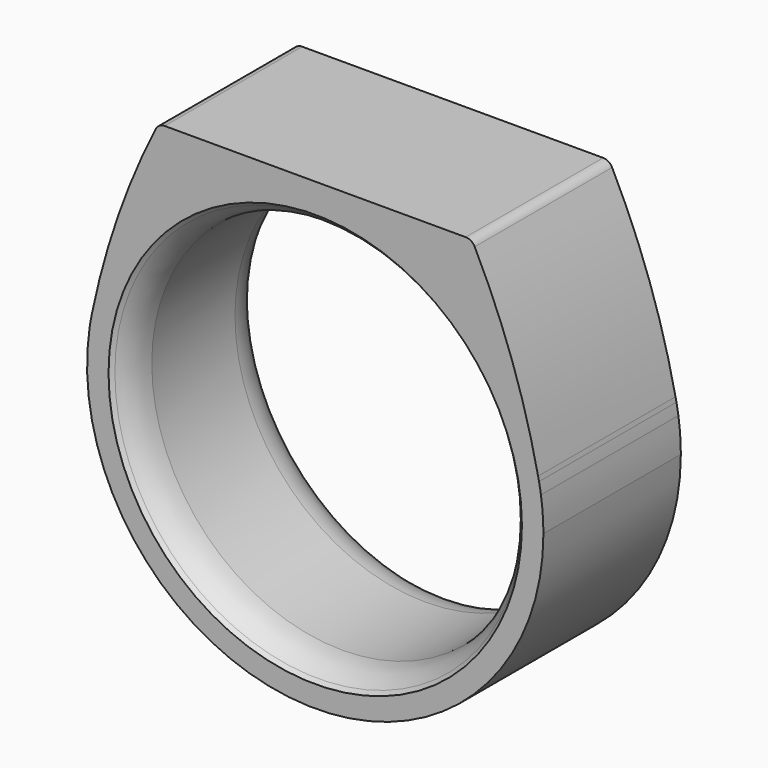
from build123d import *

# Parameters (mm, degrees)
F0_R          = 8.875
F1_DEPTH      = 4
F1_DEPTH_BACK = 4
F2_T1_DEPTH   = 10.0420034221
F3_SIZE       = 0.75
F4_R          = 0.4704417071


# Not quite as in the source:
# - a fillet or chamfer that OpenCascade refuses, or shapes differently, is made with other operations: its cross-section is extruded or revolved along the edge and cut away or added


with BuildPart() as f1:
    # F0 (on Front) → F1 (new body, two sides)
    with BuildSketch(Plane.XZ) as f1_sk:
        with BuildLine():
            ThreePointArc((-10.4432812291, 1.9566558639), (-0.9825380249, -10.5794727671), (10.625, 0))
            ThreePointArc((10.625, 0), (10.5794727671, 0.9825380249), (10.4432812291, 1.9566558639))
            ThreePointArc((10.4432812291, 1.9566558639), (10.4107043639, 2.1187258688), (10.3773464915, 2.2806369277))
            ThreePointArc((10.3773464915, 2.2806369277), (0, 10.625), (-10.3773464915, 2.2806369277))
            ThreePointArc((-10.3773464915, 2.2806369277), (-10.4107043639, 2.1187258688), (-10.4432812291, 1.9566558639))
        make_face()
        Circle(F0_R, mode=Mode.SUBTRACT)
        with BuildLine():
            ThreePointArc((-10.3773464915, 2.2806369277), (0, 10.625), (10.3773464915, 2.2806369277))
            ThreePointArc((10.3773464915, 2.2806369277), (9.1298481014, 6.734538497), (7.2942513551, 10.9800156206))
            Line((7.2942513551, 10.9800156206), (0, 10.9800156206))
            Line((0, 10.9800156206), (-7.2942513551, 10.9800156206))
            ThreePointArc((-7.2942513551, 10.9800156206), (-9.1298481014, 6.734538497), (-10.3773464915, 2.2806369277))
        make_face()
    extrude(amount=F1_DEPTH)
    extrude(f1_sk.sketch, amount=-F1_DEPTH_BACK)

    # F2: fillet of radius 10 on 2 edges, made by hand

    # F2_s2 → F2_t1 (cut)
    with BuildSketch(Plane.XZ.offset(-5.021001711)):
        with BuildLine():
            ThreePointArc((-10.5107619586, 1.5538687363), (-10.4688734573, 1.813557001), (-10.4201690702, 2.0720536626))
            ThreePointArc((-10.4201690702, 2.0720536626), (-10.4317746612, 2.0143646795), (-10.4432812291, 1.9566558639))
            ThreePointArc((-10.4432812291, 1.9566558639), (-10.4789570495, 1.7555865557), (-10.5107619586, 1.5538687363))
        make_face()
        with BuildLine():
            ThreePointArc((10.5107619586, 1.5538687363), (10.4688734573, 1.813557001), (10.4201690702, 2.0720536626))
            ThreePointArc((10.4201690702, 2.0720536626), (10.4317746612, 2.0143646795), (10.4432812291, 1.9566558639))
            ThreePointArc((10.4432812291, 1.9566558639), (10.4789570495, 1.7555865557), (10.5107619586, 1.5538687363))
        make_face()
    extrude(amount=F2_T1_DEPTH, mode=Mode.SUBTRACT)

    # F3
    f3_edges = [f1.edges().sort_by_distance(p)[0] for p in [
        (-8.875, 4, 0),
        (-8.875, -4, 0),
    ]]
    chamfer(f3_edges, length=F3_SIZE)

    # F4
    f4_edges = [f1.edges().sort_by_distance(p)[0] for p in [
        (-7.294251, 0, 10.980016),
        (7.294251, 0, 10.980016),
    ]]
    fillet(f4_edges, radius=F4_R)

    # F5: fillet of radius 2 on 2 edges, made by hand

    # F5_s1 → F5_t2 (revolve, cut)
    with BuildSketch(Plane.XY):
        with BuildLine():
            add(Edge.make_bspline(
                [(8.875, -2.4215728753), (8.875, -3.25), (9.4607864376, -3.8357864376)],
                knots=[0, 0, 0, 1, 1, 1], degree=2, weights=[1, 1, 1]))
            Line((9.4607864376, -3.8357864376), (8.875, -3.25))
            Line((8.875, -3.25), (8.875, -2.4215728753))
        make_face()
    revolve(axis=Axis((0, -3.25, 0), (0, -1, 0)), mode=Mode.SUBTRACT)

    # F5_s3 → F5_t4 (revolve, cut)
    with BuildSketch(Plane.XY):
        with BuildLine():
            add(Edge.make_bspline(
                [(9.4607864376, 3.8357864376), (8.875, 3.25), (8.875, 2.4215728753)],
                knots=[0, 0, 0, 1, 1, 1], degree=2, weights=[1, 1, 1]))
            Line((8.875, 2.4215728753), (8.875, 3.25))
            Line((8.875, 3.25), (9.4607864376, 3.8357864376))
        make_face()
    revolve(axis=Axis((0, 3.25, 0), (0, -1, 0)), mode=Mode.SUBTRACT)


solid = f1.part
